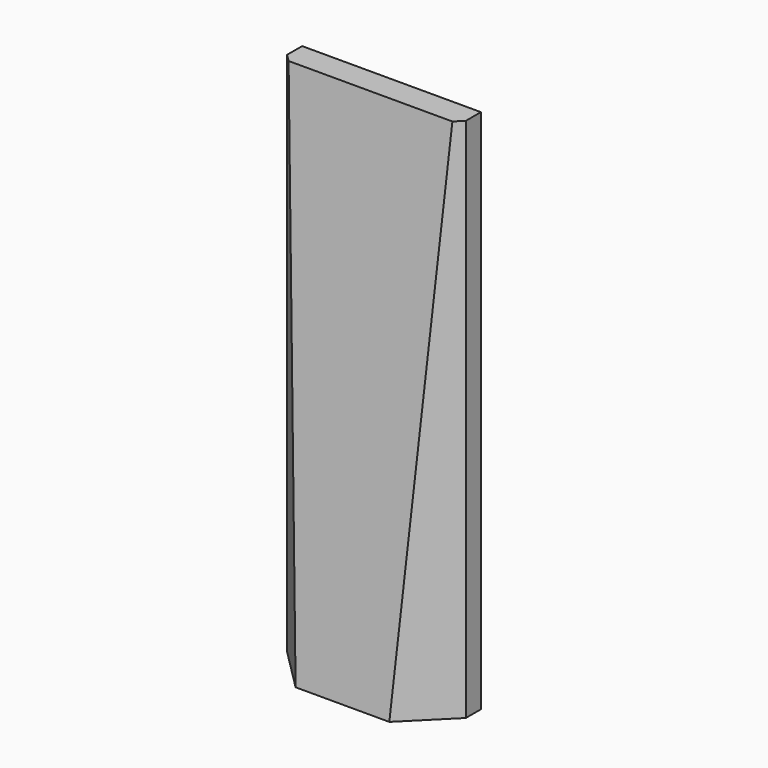
from build123d import *

# Parameters (mm, degrees)
F1_DEPTH = 30
F2_SIZE2 = 1.99999
F2_SIZE  = 29.99999


# Not quite as in the source:
# - a fillet or chamfer is up to 0.001 mm smaller than in the source, because OpenCascade refuses the exact size


with BuildPart() as f1:
    # F0 (on Top) → F1 (new body)
    with BuildSketch(Plane.XY):
        Polygon((-10.6, -0.4), (-10.6, -1.4736544004), (-8.1736544004, -3.9), (-2.8263455996, -3.9), (-0.4, -1.4736544004), (-0.4, -0.4), align=None)
    extrude(amount=F1_DEPTH)

    # F2 (size 30 and 2 in the source; OpenCascade refuses exactly that, so slightly less here)
    f2_edges = [f1.edges().sort_by_distance(p)[0] for p in [
        (-5.5, -3.9, 30),
    ]]
    f2_side = f1.faces().sort_by_distance((-5.5, -3.9, 15))[0]
    chamfer(f2_edges, length=F2_SIZE, length2=F2_SIZE2, reference=f2_side)


solid = f1.part
